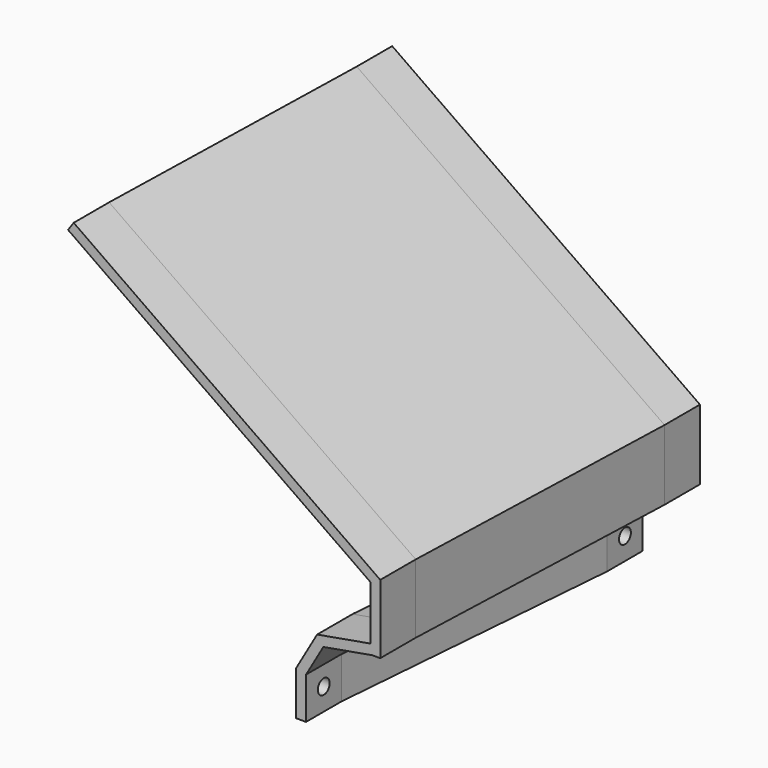
from build123d import *

# Parameters (mm, degrees)
F3_W           = 18
F3_H           = 18
F3_R           = 3
F4_DEPTH       = 2
F5_W           = 18
F5_H           = 18
F5_R           = 3
F6_DEPTH       = 2
F8_DEPTH       = 9
F8_DEPTH_BACK  = 9
F10_DEPTH      = 9
F10_DEPTH_BACK = 9
F12_DEPTH      = 18
F14_DEPTH      = 18


with BuildPart() as f4:
    # F3 (on Right) → F4 (new body, symmetric)
    with BuildSketch(Plane.YZ):
        with Locations((70.25, 0)):
            Rectangle(F3_W, F3_H)
        with Locations((70.25, 0)):
            Circle(F3_R, mode=Mode.SUBTRACT)
    extrude(amount=F4_DEPTH, both=True)

    # F7 (on offset) → F8 (join, two sides)
    with BuildSketch(Plane.XZ.offset(-70.25)) as f8_sk:
        Polygon((6.5, 23.7224318643), (-2, 9), (2, 9), (2, 7.9282032303), (9.0314862988, 20.1070947526), (21.9667090059, 22.3879235173), (21.2721162952, 26.3271545293), align=None)
    extrude(amount=-F8_DEPTH)
    extrude(f8_sk.sketch, amount=F8_DEPTH_BACK)

    # F11 (on face) → F12 (join, through all)
    with BuildSketch(Plane(origin=(0, 79.25, 0), x_dir=(-1, 0, 0), z_dir=(0, 1, 0))):
        Polygon((-21.9667090059, 22.3879235173), (-21.2721162952, 26.3271545293), (-21.2721162952, 48.8271545293), (101.6006903482, 134.863619982), (99.7962957674, 138.4832676497), (-25.2721162952, 50.9094227315), (-25.2721162952, 22.3879235173), align=None)
    extrude(amount=-F12_DEPTH)



with BuildPart() as f6:
    # F5 (on offset) → F6 (new body, symmetric)
    with BuildSketch(Plane.YZ.offset(-10)):
        with Locations((-70.25, 0)):
            Rectangle(F5_W, F5_H)
        with Locations((-70.25, 0)):
            Circle(F5_R, mode=Mode.SUBTRACT)
    extrude(amount=F6_DEPTH, both=True)

    # F9 (on offset) → F10 (join, two sides)
    with BuildSketch(Plane.XZ.offset(70.25)) as f10_sk:
        Polygon((18.1657705663, 27.542691773), (-3.5, 23.7224318643), (-12, 9), (-8, 9), (-8, 7.9282032303), (-0.9685137012, 20.1070947526), (18.8603632769, 23.603460761), align=None)
    extrude(amount=F10_DEPTH)
    extrude(f10_sk.sketch, amount=-F10_DEPTH_BACK)

    # F13 (on face) → F14 (join, through all)
    with BuildSketch(Plane.XZ.offset(79.25)):
        Polygon((18.1657705663, 49.542691773), (18.1657705663, 27.542691773), (18.8603632769, 23.603460761), (22.1657705663, 23.603460761), (22.1657705663, 51.6249599752), (-102.4127303317, 138.8557654028), (-104.7070360771, 135.5791572257), align=None)
    extrude(amount=-F14_DEPTH)


with BuildPart() as f4_1:
    add(f4.part)

    add(f6.part)  # F15 merges F6
    # F12_face (on face) → F15 section 0
    with BuildSketch(Plane(origin=(-21.9904596416, 61.25, 69.4287440583), x_dir=(1, 0, 0), z_dir=(0, -1, 0))):
        Polygon((19.9904596416, -60.4287440583), (19.9904596416, -78.4287440583), (23.9904596416, -78.4287440583), (23.9904596416, -61.500540828), (31.0219459404, -49.3216493057), (43.9571686475, -47.040820541), (47.2625759368, -47.040820541), (47.2625759368, -18.5193213268), (-77.8058361258, 69.0545235914), (-79.6102307066, 65.4348759237), (43.2625759368, -20.601589529), (43.2625759368, -43.101589529), (28.4904596416, -45.706312194), align=None)
    # F14_face (on face) → F15 section 1
    with BuildSketch(Plane(origin=(-25.2803198576, -61.25, 68.6471085342), x_dir=(-1, 0, 0), z_dir=(0, 1, 0))):
        Polygon((-13.2803198576, -77.6471085342), (-13.2803198576, -59.6471085342), (-21.7803198576, -44.9246766699), (-43.4460904239, -41.1044167612), (-43.4460904239, -19.1044167612), (79.4267162195, 66.9320486914), (77.1324104741, 70.2086568686), (-47.4460904239, -17.022148559), (-47.4460904239, -45.0436477733), (-44.1406831345, -45.0436477733), (-24.3118061564, -48.5400137817), (-17.2803198576, -60.7189053039), (-17.2803198576, -77.6471085342), align=None)
    loft()


solid = f4_1.part
